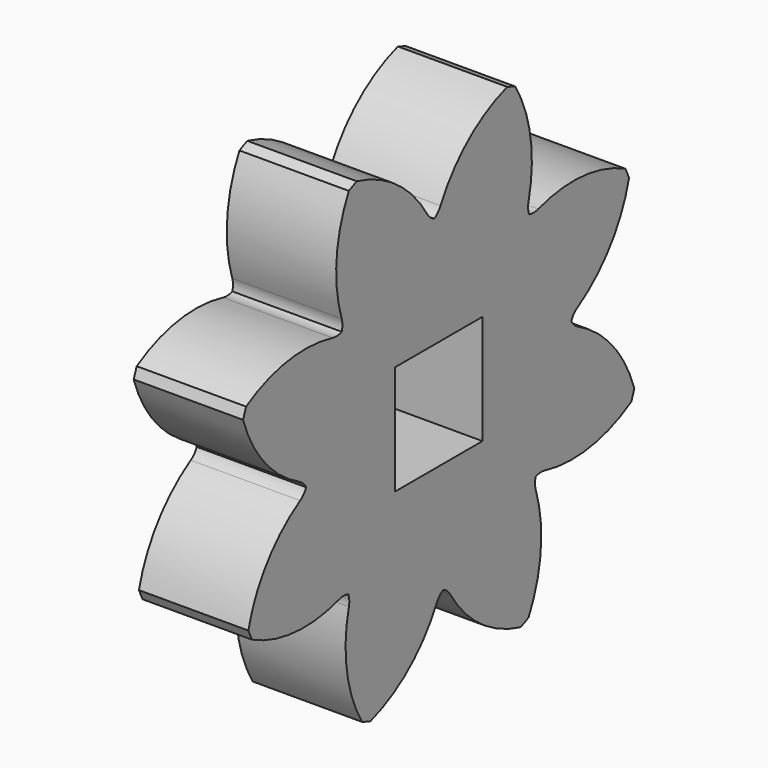
from build123d import *

# Parameters (mm, degrees)
F1_DEPTH      = 5
F2_W          = 10
F2_H          = 10
F3_DEPTH      = 5.001
F3_DEPTH_BACK = 5.001


with BuildPart() as f1:
    # F0 (on Right) → F1 (new body, symmetric)
    with BuildSketch(Plane.YZ):
        with BuildLine():
            Line((8.7534596749, 22.0049817023), (7.8275281652, 22.3511091184))
            ThreePointArc((7.8275281652, 22.3511091184), (3.3739717902, 19.8784451352), (0.2100715875, 15.8862067822))
            ThreePointArc((0.2100715875, 15.8862067822), (-0.1018352129, 15.4564251276), (-0.5296881322, 15.1418778303))
            ThreePointArc((-0.5296881322, 15.1418778303), (-0.9784750701, 15.4257588038), (-1.3196516389, 15.8326945133))
            ThreePointArc((-1.3196516389, 15.8326945133), (-4.754786797, 19.5940876069), (-9.3702410866, 21.7495024766))
            Line((-9.3702410866, 21.7495024766), (-10.2697225791, 21.3395190702))
            ThreePointArc((-10.2697225791, 21.3395190702), (-11.6704250222, 16.4419416869), (-11.084701499, 11.3817875871))
            ThreePointArc((-11.084701499, 11.3817875871), (-11.0013513902, 10.857334651), (-11.0814705639, 10.3323784235))
            ThreePointArc((-11.0814705639, 10.3323784235), (-11.5995450124, 10.2157722978), (-12.1285402775, 10.2622710322))
            ThreePointArc((-12.1285402775, 10.2622710322), (-17.2172542053, 10.4929702308), (-22.0049817023, 8.7534596749))
            Line((-22.0049817023, 8.7534596749), (-22.3511091184, 7.8275281652))
            ThreePointArc((-22.3511091184, 7.8275281652), (-19.8784451352, 3.3739717902), (-15.8862067822, 0.2100715875))
            ThreePointArc((-15.8862067822, 0.2100715875), (-15.4564251276, -0.1018352129), (-15.1418778303, -0.5296881322))
            ThreePointArc((-15.1418778303, -0.5296881322), (-15.4257588038, -0.9784750701), (-15.8326945133, -1.3196516389))
            ThreePointArc((-15.8326945133, -1.3196516389), (-19.5940876069, -4.754786797), (-21.7495024766, -9.3702410866))
            Line((-21.7495024766, -9.3702410866), (-21.3395190702, -10.2697225791))
            ThreePointArc((-21.3395190702, -10.2697225791), (-16.4419416869, -11.6704250222), (-11.3817875871, -11.084701499))
            ThreePointArc((-11.3817875871, -11.084701499), (-10.857334651, -11.0013513902), (-10.3323784235, -11.0814705639))
            ThreePointArc((-10.3323784235, -11.0814705639), (-10.2157722978, -11.5995450124), (-10.2622710322, -12.1285402775))
            ThreePointArc((-10.2622710322, -12.1285402775), (-10.4929702308, -17.2172542053), (-8.7534596749, -22.0049817023))
            Line((-8.7534596749, -22.0049817023), (-7.8275281652, -22.3511091184))
            ThreePointArc((-7.8275281652, -22.3511091184), (-3.3739717902, -19.8784451352), (-0.2100715875, -15.8862067822))
            ThreePointArc((-0.2100715875, -15.8862067822), (0.1018352129, -15.4564251276), (0.5296881322, -15.1418778303))
            ThreePointArc((0.5296881322, -15.1418778303), (0.9784750701, -15.4257588038), (1.3196516389, -15.8326945133))
            ThreePointArc((1.3196516389, -15.8326945133), (4.754786797, -19.5940876069), (9.3702410866, -21.7495024766))
            Line((9.3702410866, -21.7495024766), (10.2697225791, -21.3395190702))
            ThreePointArc((10.2697225791, -21.3395190702), (11.6704250222, -16.4419416869), (11.084701499, -11.3817875871))
            ThreePointArc((11.084701499, -11.3817875871), (11.0013513902, -10.857334651), (11.0814705639, -10.3323784235))
            ThreePointArc((11.0814705639, -10.3323784235), (11.5995450124, -10.2157722978), (12.1285402775, -10.2622710322))
            ThreePointArc((12.1285402775, -10.2622710322), (17.2172542053, -10.4929702308), (22.0049817023, -8.7534596749))
            Line((22.0049817023, -8.7534596749), (22.3511091184, -7.8275281652))
            ThreePointArc((22.3511091184, -7.8275281652), (19.8784451352, -3.3739717902), (15.8862067822, -0.2100715875))
            ThreePointArc((15.8862067822, -0.2100715875), (15.4564251276, 0.1018352129), (15.1418778303, 0.5296881322))
            ThreePointArc((15.1418778303, 0.5296881322), (15.4257588038, 0.9784750701), (15.8326945133, 1.3196516389))
            ThreePointArc((15.8326945133, 1.3196516389), (19.5940876069, 4.754786797), (21.7495024766, 9.3702410866))
            Line((21.7495024766, 9.3702410866), (21.3395190702, 10.2697225791))
            ThreePointArc((21.3395190702, 10.2697225791), (16.4419416869, 11.6704250222), (11.3817875871, 11.084701499))
            ThreePointArc((11.3817875871, 11.084701499), (10.857334651, 11.0013513902), (10.3323784235, 11.0814705639))
            ThreePointArc((10.3323784235, 11.0814705639), (10.2157722978, 11.5995450124), (10.2622710322, 12.1285402775))
            ThreePointArc((10.2622710322, 12.1285402775), (10.4929702308, 17.2172542053), (8.7534596749, 22.0049817023))
        make_face()
    extrude(amount=F1_DEPTH, both=True)

    # F2 (on Right) → F3 (cut, two sides)
    with BuildSketch(Plane.YZ) as f3_sk:
        Rectangle(F2_W, F2_H)
    extrude(amount=-F3_DEPTH, mode=Mode.SUBTRACT)
    extrude(f3_sk.sketch, amount=F3_DEPTH_BACK, mode=Mode.SUBTRACT)


solid = f1.part
